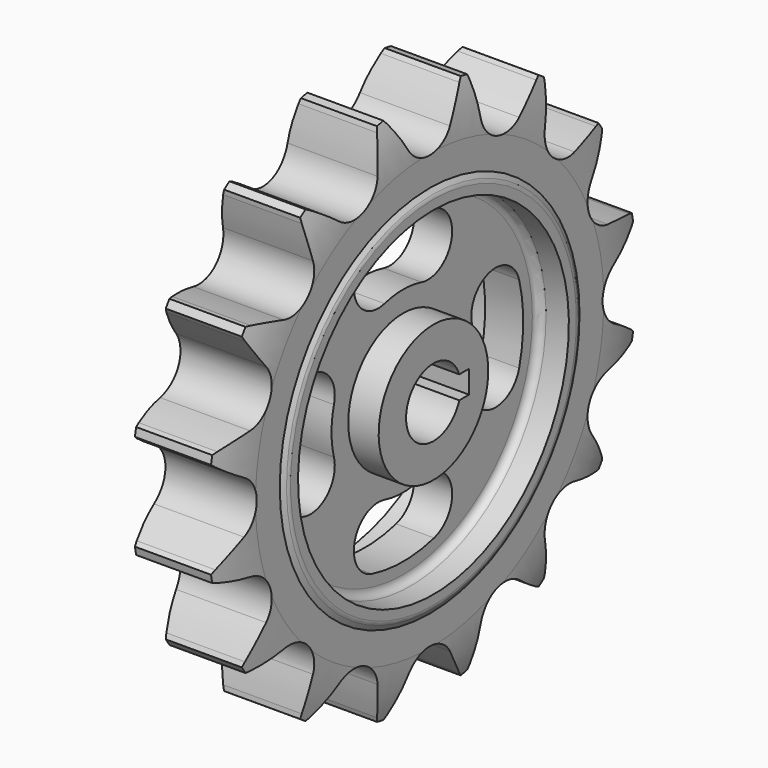
from build123d import *

# Parameters (mm, degrees)
F3_DEPTH        = 13.001
F3_DEPTH_BACK   = 13.001
F3_COPIES_COUNT = 16
F4_W            = 7.2895585008
F4_H            = 6
F5_DEPTH        = 13.001
F5_DEPTH_BACK   = 13.001
F6_R            = 2


# Not quite as in the source:
# - a pattern or mirror of a feature is missing from the dataset's text; its kind, count and spacing are read off the source's solid


with BuildPart() as f1:
    # F0 (on Front) → F1 (revolve)
    with BuildSketch(Plane.XZ):
        with BuildLine():
            Line((-13, 9), (0, 9))
            Line((0, 9), (13, 9))
            Line((13, 9), (13, 18))
            Line((13, 18), (5, 18))
            Line((5, 18), (5, 44.5))
            Line((5, 44.5), (13, 44.5))
            Line((13, 44.5), (13, 47.5))
            Line((13, 47.5), (12, 49.2487662411))
            Line((12, 49.2487662411), (12, 57.2335008386))
            ThreePointArc((12, 57.2335008386), (11.4971909226, 63.9417047711), (10, 70.5))
            Line((10, 70.5), (0, 70.5))
            Line((0, 70.5), (-10, 70.5))
            ThreePointArc((-10, 70.5), (-11.4971909226, 63.9417047711), (-12, 57.2335008386))
            Line((-12, 57.2335008386), (-12, 49.2487662411))
            Line((-12, 49.2487662411), (-13, 47.5))
            Line((-13, 47.5), (-13, 44.5))
            Line((-13, 44.5), (-5, 44.5))
            Line((-5, 44.5), (-5, 18))
            Line((-5, 18), (-13, 18))
            Line((-13, 18), (-13, 9))
        make_face()
    revolve(axis=Axis((0, 0, 0), (1, 0, 0)))

    # F2 (on Right) → F3 (cut, two sides)
    with BuildSketch(Plane.YZ) as f3_sk:
        with BuildLine():
            ThreePointArc((-11.8605483695, 68.3416372651), (-9.2548896934, 64.6355923709), (-6.8740766425, 60.78125))
            ThreePointArc((-6.8740766425, 60.78125), (0, 56.8125), (6.8740766425, 60.78125))
            ThreePointArc((6.8740766425, 60.78125), (9.2548896934, 64.6355923709), (11.8605483695, 68.3416372651))
            ThreePointArc((11.8605483695, 68.3416372651), (12.2670438809, 68.8553831196), (12.7005304186, 69.346568243))
            ThreePointArc((12.7005304186, 69.346568243), (0, 70.5), (-12.7005304186, 69.346568243))
            ThreePointArc((-12.7005304186, 69.346568243), (-12.2670438809, 68.8553831196), (-11.8605483695, 68.3416372651))
        make_face()
    f3 = extrude(amount=-F3_DEPTH, mode=Mode.SUBTRACT) + extrude(f3_sk.sketch, amount=F3_DEPTH_BACK, mode=Mode.SUBTRACT)

    # F3_copies: F3 ×16 about axis
    f3_copies_axis = Axis((0, 0, 0), (1, 0, 0))
    for i in range(1, F3_COPIES_COUNT):
        add(f3.rotate(f3_copies_axis, i * 360 / F3_COPIES_COUNT), mode=Mode.SUBTRACT)

    # F4 (on Right) → F5 (cut, two sides)
    with BuildSketch(Plane.YZ) as f5_sk:
        with Locations((8.0552207496, 0)):
            Rectangle(F4_W, F4_H)
        with BuildLine():
            ThreePointArc((-22.6992569178, -6.0822475599), (-23.5, 0), (-22.6992569178, 6.0822475599))
            ThreePointArc((-22.6992569178, 6.0822475599), (-28.3561111673, 15.880206531), (-38.1540701384, 10.2233522815))
            ThreePointArc((-38.1540701384, 10.2233522815), (-39.5, 0), (-38.1540701384, -10.2233522815))
            ThreePointArc((-38.1540701384, -10.2233522815), (-28.3561111673, -15.880206531), (-22.6992569178, -6.0822475599))
        make_face()
        with BuildLine():
            ThreePointArc((6.0822475599, -22.6992569178), (0, -23.5), (-6.0822475599, -22.6992569178))
            ThreePointArc((-6.0822475599, -22.6992569178), (-15.880206531, -28.3561111673), (-10.2233522815, -38.1540701384))
            ThreePointArc((-10.2233522815, -38.1540701384), (0, -39.5), (10.2233522815, -38.1540701384))
            ThreePointArc((10.2233522815, -38.1540701384), (15.880206531, -28.3561111673), (6.0822475599, -22.6992569178))
        make_face()
        with BuildLine():
            ThreePointArc((22.6992569178, 6.0822475599), (23.5, 0), (22.6992569178, -6.0822475599))
            ThreePointArc((22.6992569178, -6.0822475599), (28.3561111673, -15.880206531), (38.1540701384, -10.2233522815))
            ThreePointArc((38.1540701384, -10.2233522815), (39.5, 0), (38.1540701384, 10.2233522815))
            ThreePointArc((38.1540701384, 10.2233522815), (28.3561111673, 15.880206531), (22.6992569178, 6.0822475599))
        make_face()
        with BuildLine():
            ThreePointArc((-6.0822475599, 22.6992569178), (0, 23.5), (6.0822475599, 22.6992569178))
            ThreePointArc((6.0822475599, 22.6992569178), (15.880206531, 28.3561111673), (10.2233522815, 38.1540701384))
            ThreePointArc((10.2233522815, 38.1540701384), (0, 39.5), (-10.2233522815, 38.1540701384))
            ThreePointArc((-10.2233522815, 38.1540701384), (-15.880206531, 28.3561111673), (-6.0822475599, 22.6992569178))
        make_face()
    extrude(amount=-F5_DEPTH, mode=Mode.SUBTRACT)
    extrude(f5_sk.sketch, amount=F5_DEPTH_BACK, mode=Mode.SUBTRACT)

    # F6
    f6_edges = [f1.edges().sort_by_distance(p)[0] for p in [
        (5, 0, -44.5),
        (13, 0, -47.5),
    ]]
    fillet(f6_edges, radius=F6_R)


solid = f1.part
